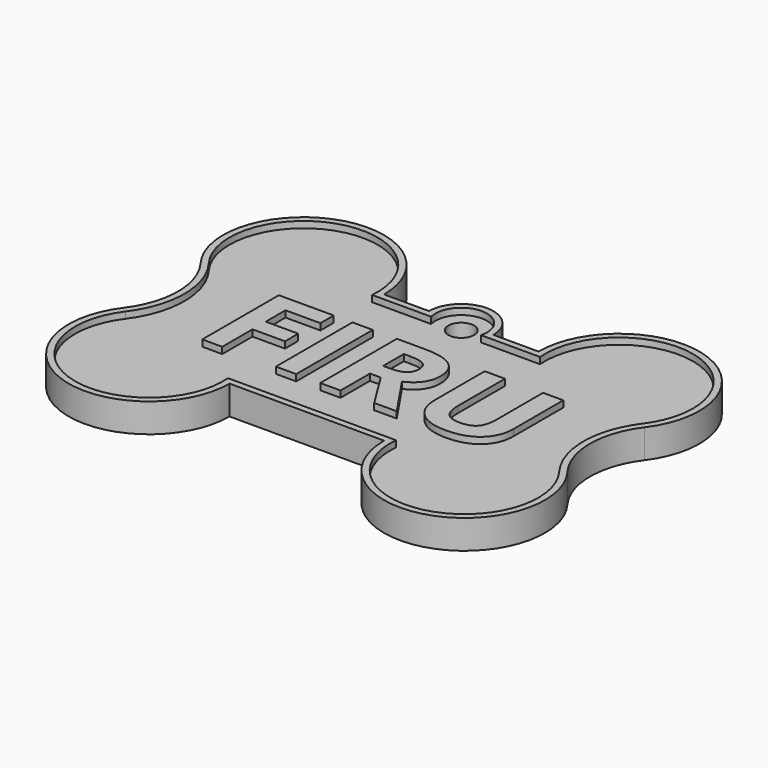
from build123d import *

# Parameters (mm, degrees)
F0_R         = 2
F1_DEPTH     = 3.5
F2_TEXT_SIZE = 20.8333333333
F3_DEPTH     = 1


# Not quite as in the source:
# - Text() gives the source's letters only with a copy of the font that has no kerning and outlines rounded to 1/6400 em; it was checked with that copy


with BuildPart() as f1:
    # F0 (on Top) → F1 (new body)
    with BuildSketch(Plane.XY):
        with BuildLine():
            Line((29.5, 30), (22.5, 30))
            ThreePointArc((22.5, 30), (6.0471529248, 41.8585412256), (0, 22.5))
            ThreePointArc((0, 22.5), (2.5, 15), (0, 7.5))
            ThreePointArc((0, 7.5), (6.0471529248, -11.8585412256), (22.5, 0))
            Line((22.5, 0), (46.5, 0))
            ThreePointArc((46.5, 0), (62.9528470752, -11.8585412256), (69, 7.5))
            ThreePointArc((69, 7.5), (66.5, 15), (69, 22.5))
            ThreePointArc((69, 22.5), (62.9528470752, 41.8585412256), (46.5, 30))
            Line((46.5, 30), (39.5, 30))
            ThreePointArc((39.5, 30), (34.5, 35), (29.5, 30))
        make_face()
        with Locations((34.5, 30)):
            Circle(F0_R, mode=Mode.SUBTRACT)
    extrude(amount=F1_DEPTH)

    # F2 (on face) → F3 (join)
    with BuildSketch(Plane.XY.offset(3.5)):
        with BuildLine():
            ThreePointArc((69, 22.5), (62.9528470752, 41.8585412256), (46.5, 30))
            Line((46.5, 30), (39.5, 30))
            ThreePointArc((39.5, 30), (34.5, 35), (29.5, 30))
            Line((29.5, 30), (22.5, 30))
            ThreePointArc((22.5, 30), (6.0471529248, 41.8585412256), (0, 22.5))
            ThreePointArc((0, 22.5), (2.5, 15), (0, 7.5))
            ThreePointArc((0, 7.5), (6.0471529248, -11.8585412256), (22.5, 0))
            Line((22.5, 0), (46.5, 0))
            ThreePointArc((46.5, 0), (62.9528470752, -11.8585412256), (69, 7.5))
            ThreePointArc((69, 7.5), (66.5, 15), (69, 22.5))
        make_face()
        with BuildLine():
            ThreePointArc((68.1999989033, 6.8999991775), (62.1583813239, -11.057784402), (47.5435622584, 1.0000013709))
            Line((47.5435622584, 1.0000013709), (21.4564377416, 1.0000013709))
            ThreePointArc((21.4564377416, 1.0000013709), (6.8416186761, -11.057784402), (0.8000010967, 6.8999991775))
            ThreePointArc((0.8000010967, 6.8999991775), (3.5000013709, 15), (0.8000010967, 23.1000008225))
            ThreePointArc((0.8000010967, 23.1000008225), (6.8416186761, 41.057784402), (21.4564377416, 28.9999986291))
            Line((21.4564377416, 28.9999986291), (30.6270184236, 28.9999986291))
            ThreePointArc((30.6270184236, 28.9999986291), (34.5, 33.9999986291), (38.3729815764, 28.9999986291))
            Line((38.3729815764, 28.9999986291), (47.5435622584, 28.9999986291))
            ThreePointArc((47.5435622584, 28.9999986291), (62.1583813239, 41.057784402), (68.1999989033, 23.1000008225))
            ThreePointArc((68.1999989033, 23.1000008225), (65.4999986291, 15), (68.1999989033, 6.8999991775))
        make_face(mode=Mode.SUBTRACT)
        with Locations((10.7923177083, 7)):
            Text('FIRU', F2_TEXT_SIZE, font='Open Sans', font_style=FontStyle.BOLD, text_align=(TextAlign.LEFT, TextAlign.BOTTOM))
    extrude(amount=F3_DEPTH)


solid = f1.part
